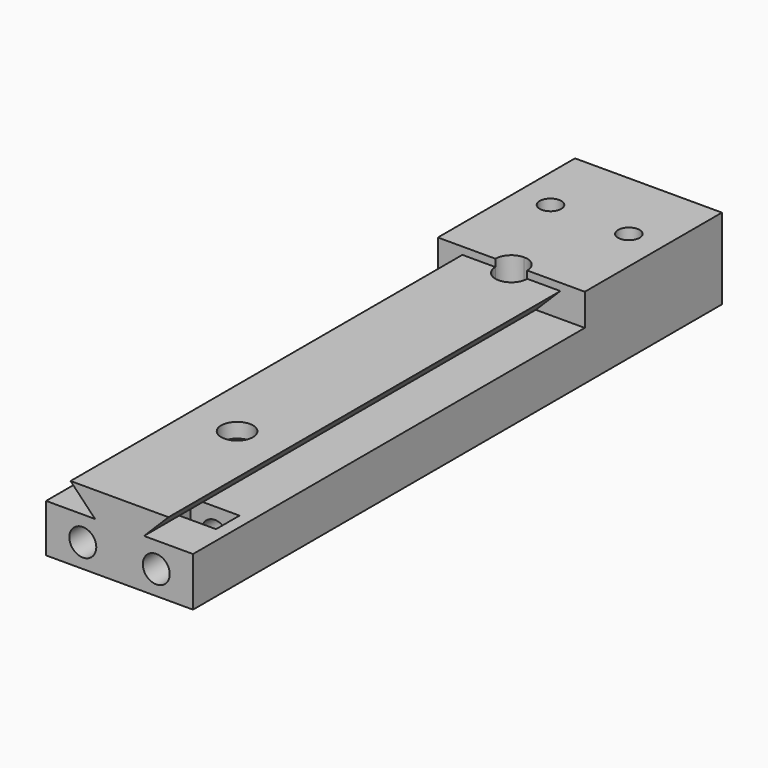
from build123d import *

# Parameters (mm, degrees)
F0_R            = 2.5000000706
F0_R_2          = 2.5000000298
F1_DEPTH        = 100
F3_DEPTH        = 35
F6_D            = 4.4
F6_DEPTH        = 40
F6_TIP          = 1.3218933619
F5_W            = 10
F5_H            = 6
F7_DEPTH        = 10
F9_D            = 5.5
F9_DEPTH        = 40
F9_TIP          = 1.6523667023
F10_DEPTH       = 4
F12_D           = 3.3
F12_CBORE_D     = 6.5
F12_CBORE_DEPTH = 3
F14_DEPTH       = 5


# Not quite as in the source:
# - ends of sketch curves that miss each other by under 0.0002 mm in the source are joined
# - a feature names something its author has since deleted; it is built from what else it names


with BuildPart() as f1:
    # F0 (on Front) → F1 (new body)
    with BuildSketch(Plane.XZ):
        Polygon((-39.8704047501, 4.2457092745), (-39.8704047501, -5.5542903855), (-9.8704054207, -5.5542903855), (-9.8704054207, 4.4457092745), (-19.8704054207, 4.4457092745), (-14.8704054207, 9.4457092745), (-24.8704050854, 9.4457092745), (-34.8704047501, 9.4457092745), (-29.8704047501, 4.2457092745), align=None)
        with Locations((-32.3704050442, -0.7542907016)):
            Circle(F0_R, mode=Mode.SUBTRACT)
        with Locations((-17.3704050202, -0.7062930843)):
            Circle(F0_R_2, mode=Mode.SUBTRACT)
        with Locations((-32.3704050442, -0.7542907016)):
            Circle(F0_R)
        with Locations((-17.3704050202, -0.7062930843)):
            Circle(F0_R_2)
    extrude(amount=F1_DEPTH)

    # F2 (on face) → F3 (join)
    with BuildSketch(Plane(origin=(0, 0, 0), x_dir=(-1, 0, 0), z_dir=(0, 1, 0))):
        Polygon((9.8704054207, 4.4457092745), (9.8704054207, -5.5542903855), (39.8704054207, -5.5542903855), (39.8704054207, 4.2457092745), (29.8704047501, 4.2457092745), (34.8704047501, 9.4457092745), (14.8704054207, 9.4457092745), (19.8704054207, 4.4457092745), align=None)
        Polygon((9.8704054207, 10.9457096145), (9.8704054207, 4.4457092745), (19.8704054207, 4.4457092745), (14.8704054207, 9.4457092745), (34.8704047501, 9.4457092745), (29.8704047501, 4.2457092745), (39.8704047501, 4.2457092745), (39.8704054207, 10.9457096145), align=None)
    extrude(amount=F3_DEPTH)

    # F4: union 

    # F6
    with Locations(Plane(origin=(0, 0, -5.5542903855), x_dir=(1, 0, 0), z_dir=(0, 0, -1))):
        with Locations((-16.8704054207, -20), (-32.8704047501, -20)):
            Hole(F6_D / 2, depth=F6_DEPTH)
            with Locations((0, 0, -(F6_DEPTH + F6_TIP / 2))):  # 118° drill point
                Cone(0, F6_D / 2, F6_TIP, mode=Mode.SUBTRACT)

    # F5 (on face) → F7 (cut)
    with BuildSketch(Plane(origin=(0, 0, -5.5542903855), x_dir=(1, 0, 0), z_dir=(0, 0, -1))):
        with Locations((-17.3704054207, 88)):
            Rectangle(F5_W, F5_H)
        with Locations((-32.3704047501, 88)):
            Rectangle(F5_W, F5_H)
    extrude(amount=-F7_DEPTH, mode=Mode.SUBTRACT)

    # F9
    with Locations(Plane.XZ.offset(100)):
        with Locations((-32.3704050442, -0.7542907016), (-17.3704050202, -0.7062930843)):
            Hole(F9_D / 2, depth=F9_DEPTH)
            with Locations((0, 0, -(F9_DEPTH + F9_TIP / 2))):  # 118° drill point
                Cone(0, F9_D / 2, F9_TIP, mode=Mode.SUBTRACT)

    # F5 (on face) → F10 (cut)
    with BuildSketch(Plane(origin=(0, 0, -5.5542903855), x_dir=(1, 0, 0), z_dir=(0, 0, -1))):
        Polygon((-20.3704054207, -17.9792740578), (-20.3704054207, -22.0207259422), (-16.8704054207, -24.0414518843), (-13.3704054207, -22.0207259422), (-13.3704054207, -17.9792740578), (-16.8704054207, -15.9585481157), align=None)
        Polygon((-32.7971248335, -24.0407874712), (-29.3343401905, -21.9569314662), (-29.4076201071, -17.9161439951), (-32.9436846667, -15.9592125288), (-36.4064693097, -18.0430685338), (-36.3331893931, -22.0838560049), align=None)
    extrude(amount=-F10_DEPTH, mode=Mode.SUBTRACT)

    # F12 (through all)
    with Locations(Plane.XY.offset(9.4457092745)):
        with Locations((-24.8704050854, 0), (-24.8704050854, -70)):
            CounterBoreHole(F12_D / 2, F12_CBORE_D / 2, F12_CBORE_DEPTH)

    # F13 (on face) → F14 (cut)
    with BuildSketch(Plane.XY.offset(10.9457096145)):
        with BuildLine():
            Line((-28.1204054207, 0), (-21.6204054207, 0))
            ThreePointArc((-21.6204054207, 0), (-24.8704054207, 3.25), (-28.1204054207, 0))
        make_face()
    extrude(amount=-F14_DEPTH, mode=Mode.SUBTRACT)


solid = f1.part
